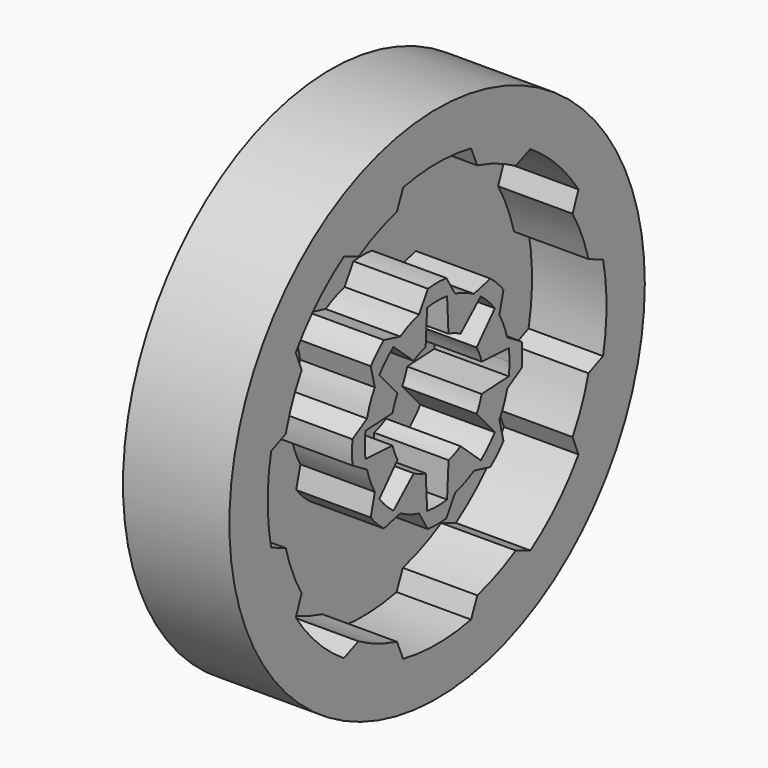
from build123d import *

# Parameters (mm, degrees)
F3_DEPTH = 35
F6_DEPTH = 35
F7_R     = 116.5
F7_R_2   = 99.5
F8_DEPTH = 35


# Not quite as in the source:
# - a feature names something its author has since deleted; it is built from what else it names


with BuildPart() as f1:
    # F0 (on Top) → F1 (revolve)
    with BuildSketch(Plane.XY):
        Polygon((-35, 92), (0, 92), (0, 122), (-50, 122), (-50, 0), (-35, 0), align=None)
    revolve(axis=Axis((-42.5, 0, 0), (1, 0, 0)))

    # F2 (on face) → F3 (cut)
    with BuildSketch(Plane.YZ):
        with BuildLine():
            ThreePointArc((-23.6019687167, 88.9210159225), (0, 92), (23.6019687167, 88.9210159225))
            Line((23.6019687167, 88.9210159225), (19.9614730536, 97.4771234369))
            ThreePointArc((19.9614730536, 97.4771234369), (0, 99.5), (-19.9614730536, 97.4771234369))
            Line((-19.9614730536, 97.4771234369), (-23.6019687167, 88.9210159225))
        make_face()
        with BuildLine():
            ThreePointArc((-19.9614730536, 97.4771234369), (0, 99.5), (19.9614730536, 97.4771234369))
            Line((19.9614730536, 97.4771234369), (12.8102793756, 114.2842803815))
            ThreePointArc((12.8102793756, 114.2842803815), (0, 115), (-12.8102793756, 114.2842803815))
            Line((-12.8102793756, 114.2842803815), (-19.9614730536, 97.4771234369))
        make_face()
        with BuildLine():
            ThreePointArc((-79.5657654778, 46.1875412199), (-65.0538238692, 65.0538238692), (-46.1875412199, 79.5657654778))
            Line((-46.1875412199, 79.5657654778), (-54.8118420341, 83.0416279515))
            ThreePointArc((-54.8118420341, 83.0416279515), (-70.3571247281, 70.3571247281), (-83.0416279515, 54.8118420341))
            Line((-83.0416279515, 54.8118420341), (-79.5657654778, 46.1875412199))
        make_face()
        with BuildLine():
            ThreePointArc((-83.0416279515, 54.8118420341), (-70.3571247281, 70.3571247281), (-54.8118420341, 83.0416279515))
            Line((-54.8118420341, 83.0416279515), (-71.7529542254, 89.8694250562))
            ThreePointArc((-71.7529542254, 89.8694250562), (-81.3172798365, 81.3172798365), (-89.8694250562, 71.7529542254))
            Line((-89.8694250562, 71.7529542254), (-83.0416279515, 54.8118420341))
        make_face()
        with BuildLine():
            ThreePointArc((-88.9210159225, -23.6019687167), (-92, 0), (-88.9210159225, 23.6019687167))
            Line((-88.9210159225, 23.6019687167), (-97.4771234369, 19.9614730536))
            ThreePointArc((-97.4771234369, 19.9614730536), (-99.5, 0), (-97.4771234369, -19.9614730536))
            Line((-97.4771234369, -19.9614730536), (-88.9210159225, -23.6019687167))
        make_face()
        with BuildLine():
            ThreePointArc((-97.4771234369, -19.9614730536), (-99.5, 0), (-97.4771234369, 19.9614730536))
            Line((-97.4771234369, 19.9614730536), (-114.2842803815, 12.8102793756))
            ThreePointArc((-114.2842803815, 12.8102793756), (-115, 0), (-114.2842803815, -12.8102793756))
            Line((-114.2842803815, -12.8102793756), (-97.4771234369, -19.9614730536))
        make_face()
        with BuildLine():
            ThreePointArc((-46.1875412199, -79.5657654778), (-65.0538238692, -65.0538238692), (-79.5657654778, -46.1875412199))
            Line((-79.5657654778, -46.1875412199), (-83.0416279515, -54.8118420341))
            ThreePointArc((-83.0416279515, -54.8118420341), (-70.3571247281, -70.3571247281), (-54.8118420341, -83.0416279515))
            Line((-54.8118420341, -83.0416279515), (-46.1875412199, -79.5657654778))
        make_face()
        with BuildLine():
            ThreePointArc((-54.8118420341, -83.0416279515), (-70.3571247281, -70.3571247281), (-83.0416279515, -54.8118420341))
            Line((-83.0416279515, -54.8118420341), (-89.8694250562, -71.7529542254))
            ThreePointArc((-89.8694250562, -71.7529542254), (-81.3172798365, -81.3172798365), (-71.7529542254, -89.8694250562))
            Line((-71.7529542254, -89.8694250562), (-54.8118420341, -83.0416279515))
        make_face()
        with BuildLine():
            Line((19.9614730536, -97.4771234369), (23.6019687167, -88.9210159225))
            ThreePointArc((23.6019687167, -88.9210159225), (0, -92), (-23.6019687167, -88.9210159225))
            Line((-23.6019687167, -88.9210159225), (-19.9614730536, -97.4771234369))
            ThreePointArc((-19.9614730536, -97.4771234369), (0, -99.5), (19.9614730536, -97.4771234369))
        make_face()
        with BuildLine():
            Line((12.8102793756, -114.2842803815), (19.9614730536, -97.4771234369))
            ThreePointArc((19.9614730536, -97.4771234369), (0, -99.5), (-19.9614730536, -97.4771234369))
            Line((-19.9614730536, -97.4771234369), (-12.8102793756, -114.2842803815))
            ThreePointArc((-12.8102793756, -114.2842803815), (0, -115), (12.8102793756, -114.2842803815))
        make_face()
        with BuildLine():
            Line((83.0416279515, -54.8118420341), (79.5657654778, -46.1875412199))
            ThreePointArc((79.5657654778, -46.1875412199), (65.0538238692, -65.0538238692), (46.1875412199, -79.5657654778))
            Line((46.1875412199, -79.5657654778), (54.8118420341, -83.0416279515))
            ThreePointArc((54.8118420341, -83.0416279515), (70.3571247281, -70.3571247281), (83.0416279515, -54.8118420341))
        make_face()
        with BuildLine():
            Line((89.8694250562, -71.7529542254), (83.0416279515, -54.8118420341))
            ThreePointArc((83.0416279515, -54.8118420341), (70.3571247281, -70.3571247281), (54.8118420341, -83.0416279515))
            Line((54.8118420341, -83.0416279515), (71.7529542254, -89.8694250562))
            ThreePointArc((71.7529542254, -89.8694250562), (81.3172798365, -81.3172798365), (89.8694250562, -71.7529542254))
        make_face()
        with BuildLine():
            Line((97.4771234369, 19.9614730536), (88.9210159225, 23.6019687167))
            ThreePointArc((88.9210159225, 23.6019687167), (91.2270065958, 11.9009775886), (92, 0))
            ThreePointArc((92, 0), (91.2270065958, -11.9009775886), (88.9210159225, -23.6019687167))
            Line((88.9210159225, -23.6019687167), (97.4771234369, -19.9614730536))
            ThreePointArc((97.4771234369, -19.9614730536), (98.9929891002, -10.0318547146), (99.5, 0))
            ThreePointArc((99.5, 0), (98.9929891002, 10.0318547146), (97.4771234369, 19.9614730536))
        make_face()
        with BuildLine():
            Line((114.2842803815, 12.8102793756), (97.4771234369, 19.9614730536))
            ThreePointArc((97.4771234369, 19.9614730536), (98.9929891002, 10.0318547146), (99.5, 0))
            ThreePointArc((99.5, 0), (98.9929891002, -10.0318547146), (97.4771234369, -19.9614730536))
            Line((97.4771234369, -19.9614730536), (114.2842803815, -12.8102793756))
            ThreePointArc((114.2842803815, -12.8102793756), (115, 0), (114.2842803815, 12.8102793756))
        make_face()
        with BuildLine():
            Line((54.8118420341, 83.0416279515), (46.1875412199, 79.5657654778))
            ThreePointArc((46.1875412199, 79.5657654778), (65.0538238692, 65.0538238692), (79.5657654778, 46.1875412199))
            Line((79.5657654778, 46.1875412199), (83.0416279515, 54.8118420341))
            ThreePointArc((83.0416279515, 54.8118420341), (70.3571247281, 70.3571247281), (54.8118420341, 83.0416279515))
        make_face()
        with BuildLine():
            Line((71.7529542254, 89.8694250562), (54.8118420341, 83.0416279515))
            ThreePointArc((54.8118420341, 83.0416279515), (70.3571247281, 70.3571247281), (83.0416279515, 54.8118420341))
            Line((83.0416279515, 54.8118420341), (89.8694250562, 71.7529542254))
            ThreePointArc((89.8694250562, 71.7529542254), (81.3172798365, 81.3172798365), (71.7529542254, 89.8694250562))
        make_face()
    extrude(amount=-F3_DEPTH, mode=Mode.SUBTRACT)

    # F5 (on face) → F6 (join)
    with BuildSketch(Plane.YZ.offset(-35)):
        with BuildLine():
            Line((5.8489450002, 42.0956035992), (5.452030419, 49.7018647971))
            ThreePointArc((5.452030419, 49.7018647971), (0.0155501533, 49.9999975819), (-5.4211145011, 49.7052463787))
            Line((-5.4211145011, 49.7052463787), (-5.8439419576, 42.0962984406))
            ThreePointArc((-5.8439419576, 42.0962984406), (0.0025255316, 42.499999925), (5.8489450002, 42.0956035992))
        make_face()
        with BuildLine():
            Line((10.5155718212, 41.1785471972), (5.452030419, 49.7018647971))
            Line((5.452030419, 49.7018647971), (5.8489450002, 42.0956035992))
            ThreePointArc((5.8489450002, 42.0956035992), (8.1950961441, 41.7024027987), (10.5155718212, 41.1785471972))
        make_face()
        with BuildLine():
            Line((-5.8439419576, 42.0962984406), (-5.4211145011, 49.7052463787))
            Line((-5.4211145011, 49.7052463787), (-10.5938325524, 41.1584828663))
            ThreePointArc((-10.5938325524, 41.1584828663), (-8.2322525607, 41.6950838562), (-5.8439419576, 42.0962984406))
        make_face()
        with BuildLine():
            ThreePointArc((10.5155718212, 41.1785471972), (8.1950961441, 41.7024027987), (5.8489450002, 42.0956035992))
            Line((5.8489450002, 42.0956035992), (6.6804809217, 26.1604888076))
            ThreePointArc((6.6804809217, 26.1604888076), (10.3087382214, 24.9545570244), (13.7302760127, 23.2482154286))
            Line((13.7302760127, 23.2482154286), (25.6342871031, 33.8988690772))
            ThreePointArc((25.6342871031, 33.8988690772), (23.6617949268, 35.303958147), (21.6124715015, 36.5944131746))
            ThreePointArc((21.6124715015, 36.5944131746), (16.2267175708, 39.2803212421), (10.5155718212, 41.1785471972))
        make_face()
        with BuildLine():
            Line((-6.7301995039, 26.1477420562), (-5.8439419576, 42.0962984406))
            ThreePointArc((-5.8439419576, 42.0962984406), (-8.2322525607, 41.6950838562), (-10.5938325524, 41.1584828663))
            ThreePointArc((-10.5938325524, 41.1584828663), (-16.3013594868, 39.2494035481), (-21.6819978197, 36.5532621054))
            ThreePointArc((-21.6819978197, 36.5532621054), (-23.6932437548, 35.2828598667), (-25.6302580907, 33.9019154356))
            Line((-25.6302580907, 33.9019154356), (-13.7744456737, 23.2220723964))
            ThreePointArc((-13.7744456737, 23.2220723964), (-10.3561577916, 24.9349151953), (-6.7301995039, 26.1477420562))
        make_face()
        with BuildLine():
            Line((31.3136099496, 38.9802236003), (21.6124715015, 36.5944131746))
            ThreePointArc((21.6124715015, 36.5944131746), (23.6617949268, 35.303958147), (25.6342871031, 33.8988690772))
            Line((25.6342871031, 33.8988690772), (31.3136099496, 38.9802236003))
        make_face()
        with BuildLine():
            ThreePointArc((-25.6302580907, 33.9019154356), (-23.6932437548, 35.2828598667), (-21.6819978197, 36.5532621054))
            Line((-21.6819978197, 36.5532621054), (-31.2893579551, 38.9996933162))
            Line((-31.2893579551, 38.9996933162), (-25.6302580907, 33.9019154356))
        make_face()
        with BuildLine():
            Line((31.3136099496, 38.9802236003), (25.6342871031, 33.8988690772))
            ThreePointArc((25.6342871031, 33.8988690772), (30.0538239679, 30.0502523268), (33.9019154356, 25.6302580907))
            Line((33.9019154356, 25.6302580907), (38.9996933162, 31.2893579551))
            ThreePointArc((38.9996933162, 31.2893579551), (35.3663329683, 35.3443417306), (31.3136099496, 38.9802236003))
        make_face()
        with BuildLine():
            ThreePointArc((-33.8988690772, 25.6342871031), (-30.0502523268, 30.0538239679), (-25.6302580907, 33.9019154356))
            Line((-25.6302580907, 33.9019154356), (-31.2893579551, 38.9996933162))
            ThreePointArc((-31.2893579551, 38.9996933162), (-35.3443417306, 35.3663329683), (-38.9802236003, 31.3136099496))
            Line((-38.9802236003, 31.3136099496), (-33.8988690772, 25.6342871031))
        make_face()
        with BuildLine():
            Line((33.9019154356, 25.6302580907), (23.2220723964, 13.7744456737))
            ThreePointArc((23.2220723964, 13.7744456737), (24.9349151953, 10.3561577916), (26.1477420562, 6.7301995039))
            Line((26.1477420562, 6.7301995039), (42.0962984406, 5.8439419576))
            ThreePointArc((42.0962984406, 5.8439419576), (41.6950838562, 8.2322525607), (41.1584828663, 10.5938325524))
            ThreePointArc((41.1584828663, 10.5938325524), (39.2494035481, 16.3013594868), (36.5532621054, 21.6819978197))
            ThreePointArc((36.5532621054, 21.6819978197), (35.2828598667, 23.6932437548), (33.9019154356, 25.6302580907))
        make_face()
        with BuildLine():
            Line((38.9996933162, 31.2893579551), (33.9019154356, 25.6302580907))
            ThreePointArc((33.9019154356, 25.6302580907), (35.2828598667, 23.6932437548), (36.5532621054, 21.6819978197))
            Line((36.5532621054, 21.6819978197), (38.9996933162, 31.2893579551))
        make_face()
        with BuildLine():
            ThreePointArc((-26.1604888076, 6.6804809217), (-24.9545570244, 10.3087382214), (-23.2482154286, 13.7302760127))
            Line((-23.2482154286, 13.7302760127), (-33.8988690772, 25.6342871031))
            ThreePointArc((-33.8988690772, 25.6342871031), (-35.303958147, 23.6617949268), (-36.5944131746, 21.6124715015))
            ThreePointArc((-36.5944131746, 21.6124715015), (-39.2803212421, 16.2267175708), (-41.1785471972, 10.5155718212))
            ThreePointArc((-41.1785471972, 10.5155718212), (-41.7024027987, 8.1950961441), (-42.0956035992, 5.8489450002))
            Line((-42.0956035992, 5.8489450002), (-26.1604888076, 6.6804809217))
        make_face()
        with BuildLine():
            ThreePointArc((-36.5944131746, 21.6124715015), (-35.303958147, 23.6617949268), (-33.8988690772, 25.6342871031))
            Line((-33.8988690772, 25.6342871031), (-38.9802236003, 31.3136099496))
            Line((-38.9802236003, 31.3136099496), (-36.5944131746, 21.6124715015))
        make_face()
        with BuildLine():
            ThreePointArc((41.1584828663, 10.5938325524), (41.6950838562, 8.2322525607), (42.0962984406, 5.8439419576))
            Line((42.0962984406, 5.8439419576), (49.7052463787, 5.4211145011))
            Line((49.7052463787, 5.4211145011), (41.1584828663, 10.5938325524))
        make_face()
        with BuildLine():
            Line((49.7052463787, 5.4211145011), (42.0962984406, 5.8439419576))
            ThreePointArc((42.0962984406, 5.8439419576), (42.3989544902, 2.9289346422), (42.5, 0))
            ThreePointArc((42.5, 0), (42.3987803655, -2.9314541641), (42.0956035992, -5.8489450002))
            Line((42.0956035992, -5.8489450002), (49.7018647971, -5.452030419))
            ThreePointArc((49.7018647971, -5.452030419), (49.9999975819, -0.0155501533), (49.7052463787, 5.4211145011))
        make_face()
        with BuildLine():
            ThreePointArc((-23.2220723964, -13.7744456737), (-24.9349151953, -10.3561577916), (-26.1477420562, -6.7301995039))
            Line((-26.1477420562, -6.7301995039), (-42.0962984406, -5.8439419576))
            ThreePointArc((-42.0962984406, -5.8439419576), (-41.6950838562, -8.2322525607), (-41.1584828663, -10.5938325524))
            ThreePointArc((-41.1584828663, -10.5938325524), (-39.2494035481, -16.3013594868), (-36.5532621054, -21.6819978197))
            ThreePointArc((-36.5532621054, -21.6819978197), (-35.2828598667, -23.6932437548), (-33.9019154356, -25.6302580907))
            Line((-33.9019154356, -25.6302580907), (-23.2220723964, -13.7744456737))
        make_face()
        with BuildLine():
            ThreePointArc((-42.0962984406, -5.8439419576), (-42.499999925, 0.0025255316), (-42.0956035992, 5.8489450002))
            Line((-42.0956035992, 5.8489450002), (-49.7018647971, 5.452030419))
            ThreePointArc((-49.7018647971, 5.452030419), (-49.9999975819, 0.0155501533), (-49.7052463787, -5.4211145011))
            Line((-49.7052463787, -5.4211145011), (-42.0962984406, -5.8439419576))
        make_face()
        with BuildLine():
            Line((-49.7018647971, 5.452030419), (-42.0956035992, 5.8489450002))
            ThreePointArc((-42.0956035992, 5.8489450002), (-41.7024027987, 8.1950961441), (-41.1785471972, 10.5155718212))
            Line((-41.1785471972, 10.5155718212), (-49.7018647971, 5.452030419))
        make_face()
        with BuildLine():
            Line((42.0956035992, -5.8489450002), (26.1604888076, -6.6804809217))
            ThreePointArc((26.1604888076, -6.6804809217), (24.9545570244, -10.3087382214), (23.2482154286, -13.7302760127))
            Line((23.2482154286, -13.7302760127), (33.8988690772, -25.6342871031))
            ThreePointArc((33.8988690772, -25.6342871031), (35.303958147, -23.6617949268), (36.5944131746, -21.6124715015))
            ThreePointArc((36.5944131746, -21.6124715015), (39.2803212421, -16.2267175708), (41.1785471972, -10.5155718212))
            ThreePointArc((41.1785471972, -10.5155718212), (41.7024027987, -8.1950961441), (42.0956035992, -5.8489450002))
        make_face()
        with BuildLine():
            ThreePointArc((-41.1584828663, -10.5938325524), (-41.6950838562, -8.2322525607), (-42.0962984406, -5.8439419576))
            Line((-42.0962984406, -5.8439419576), (-49.7052463787, -5.4211145011))
            Line((-49.7052463787, -5.4211145011), (-41.1584828663, -10.5938325524))
        make_face()
        with BuildLine():
            Line((49.7018647971, -5.452030419), (42.0956035992, -5.8489450002))
            ThreePointArc((42.0956035992, -5.8489450002), (41.7024027987, -8.1950961441), (41.1785471972, -10.5155718212))
            Line((41.1785471972, -10.5155718212), (49.7018647971, -5.452030419))
        make_face()
        with BuildLine():
            ThreePointArc((-6.6804809217, -26.1604888076), (-10.3087382214, -24.9545570244), (-13.7302760127, -23.2482154286))
            Line((-13.7302760127, -23.2482154286), (-25.6342871031, -33.8988690772))
            ThreePointArc((-25.6342871031, -33.8988690772), (-23.6617949268, -35.303958147), (-21.6124715015, -36.5944131746))
            ThreePointArc((-21.6124715015, -36.5944131746), (-16.2267175708, -39.2803212421), (-10.5155718212, -41.1785471972))
            ThreePointArc((-10.5155718212, -41.1785471972), (-8.1950961441, -41.7024027987), (-5.8489450002, -42.0956035992))
            Line((-5.8489450002, -42.0956035992), (-6.6804809217, -26.1604888076))
        make_face()
        with BuildLine():
            ThreePointArc((-25.6342871031, -33.8988690772), (-30.0538239679, -30.0502523268), (-33.9019154356, -25.6302580907))
            Line((-33.9019154356, -25.6302580907), (-38.9996933162, -31.2893579551))
            ThreePointArc((-38.9996933162, -31.2893579551), (-35.3663329683, -35.3443417306), (-31.3136099496, -38.9802236003))
            Line((-31.3136099496, -38.9802236003), (-25.6342871031, -33.8988690772))
        make_face()
        with BuildLine():
            Line((-38.9996933162, -31.2893579551), (-33.9019154356, -25.6302580907))
            ThreePointArc((-33.9019154356, -25.6302580907), (-35.2828598667, -23.6932437548), (-36.5532621054, -21.6819978197))
            Line((-36.5532621054, -21.6819978197), (-38.9996933162, -31.2893579551))
        make_face()
        with BuildLine():
            Line((25.6302580907, -33.9019154356), (13.7744456737, -23.2220723964))
            ThreePointArc((13.7744456737, -23.2220723964), (10.3561577916, -24.9349151953), (6.7301995039, -26.1477420562))
            Line((6.7301995039, -26.1477420562), (5.8439419576, -42.0962984406))
            ThreePointArc((5.8439419576, -42.0962984406), (8.2322525607, -41.6950838562), (10.5938325524, -41.1584828663))
            ThreePointArc((10.5938325524, -41.1584828663), (16.3013594868, -39.2494035481), (21.6819978197, -36.5532621054))
            ThreePointArc((21.6819978197, -36.5532621054), (23.6932437548, -35.2828598667), (25.6302580907, -33.9019154356))
        make_face()
        with BuildLine():
            ThreePointArc((36.5944131746, -21.6124715015), (35.303958147, -23.6617949268), (33.8988690772, -25.6342871031))
            Line((33.8988690772, -25.6342871031), (38.9802236003, -31.3136099496))
            Line((38.9802236003, -31.3136099496), (36.5944131746, -21.6124715015))
        make_face()
        with BuildLine():
            Line((38.9802236003, -31.3136099496), (33.8988690772, -25.6342871031))
            ThreePointArc((33.8988690772, -25.6342871031), (30.0502523268, -30.0538239679), (25.6302580907, -33.9019154356))
            Line((25.6302580907, -33.9019154356), (31.2893579551, -38.9996933162))
            ThreePointArc((31.2893579551, -38.9996933162), (35.3443417306, -35.3663329683), (38.9802236003, -31.3136099496))
        make_face()
        with BuildLine():
            ThreePointArc((-21.6124715015, -36.5944131746), (-23.6617949268, -35.303958147), (-25.6342871031, -33.8988690772))
            Line((-25.6342871031, -33.8988690772), (-31.3136099496, -38.9802236003))
            Line((-31.3136099496, -38.9802236003), (-21.6124715015, -36.5944131746))
        make_face()
        with BuildLine():
            Line((31.2893579551, -38.9996933162), (25.6302580907, -33.9019154356))
            ThreePointArc((25.6302580907, -33.9019154356), (23.6932437548, -35.2828598667), (21.6819978197, -36.5532621054))
            Line((21.6819978197, -36.5532621054), (31.2893579551, -38.9996933162))
        make_face()
        with BuildLine():
            ThreePointArc((5.8439419576, -42.0962984406), (-0.0025255316, -42.499999925), (-5.8489450002, -42.0956035992))
            Line((-5.8489450002, -42.0956035992), (-5.452030419, -49.7018647971))
            ThreePointArc((-5.452030419, -49.7018647971), (-0.0155501533, -49.9999975819), (5.4211145011, -49.7052463787))
            Line((5.4211145011, -49.7052463787), (5.8439419576, -42.0962984406))
        make_face()
        with BuildLine():
            Line((-5.452030419, -49.7018647971), (-5.8489450002, -42.0956035992))
            ThreePointArc((-5.8489450002, -42.0956035992), (-8.1950961441, -41.7024027987), (-10.5155718212, -41.1785471972))
            Line((-10.5155718212, -41.1785471972), (-5.452030419, -49.7018647971))
        make_face()
        with BuildLine():
            ThreePointArc((10.5938325524, -41.1584828663), (8.2322525607, -41.6950838562), (5.8439419576, -42.0962984406))
            Line((5.8439419576, -42.0962984406), (5.4211145011, -49.7052463787))
            Line((5.4211145011, -49.7052463787), (10.5938325524, -41.1584828663))
        make_face()
    extrude(amount=F6_DEPTH)

    # F7 (on face) → F8 (join)
    with BuildSketch(Plane.YZ.offset(-35)):
        Circle(F7_R)
        Circle(F7_R_2, mode=Mode.SUBTRACT)
    extrude(amount=F8_DEPTH)


solid = f1.part
